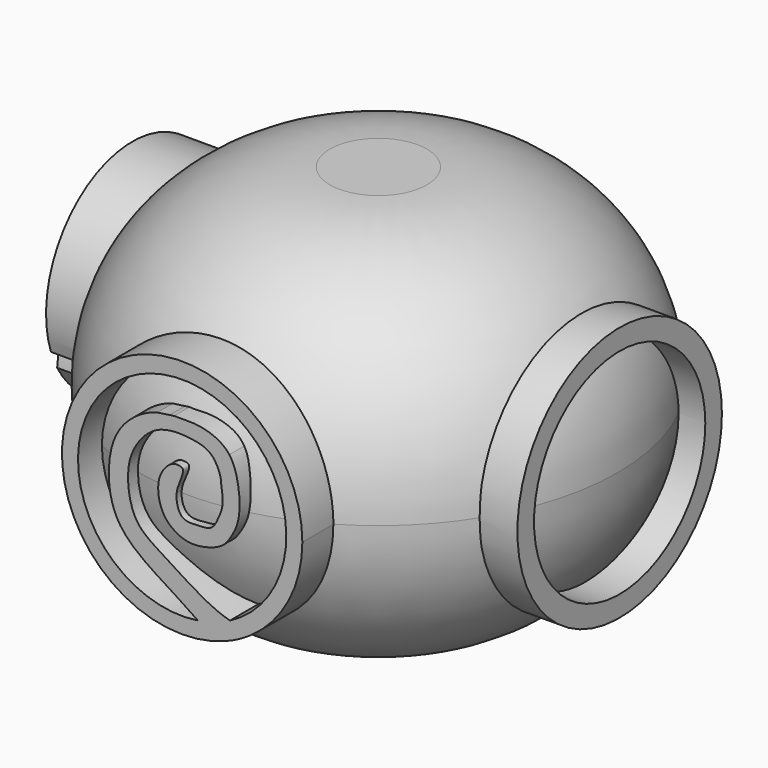
from build123d import *

# Parameters (mm, degrees)
F0_R      = 15.9252372122
F1_DEPTH  = 25.4
F2_R      = 12.69999
F5_DEPTH  = 4.826
F7_R      = 8.4966249318
F7_R_2    = 7.1160692684
F8_DEPTH  = 2.54
F11_DEPTH = 4.572


# Not quite as in the source:
# - a fillet or chamfer is up to 0.001 mm smaller than in the source, because OpenCascade refuses the exact size


with BuildPart() as f1:
    # F0 (on Top) → F1 (new body)
    with BuildSketch(Plane.XY):
        with Locations((-45.4665385187, 19.9958086014)):
            Circle(F0_R)
    extrude(amount=F1_DEPTH)

    # F2 (radius 12.7 in the source; OpenCascade refuses exactly that, so slightly less here)
    f2_edges = [f1.edges().sort_by_distance(p)[0] for p in [
        (-61.391776, 19.995809, 25.4),
        (-61.391776, 19.995809, 0),
    ]]
    fillet(f2_edges, radius=F2_R)

    # F4 (on offset) → F5 (join)
    with BuildSketch(Plane.XZ.offset(-8.4836)):
        with BuildLine():
            ThreePointArc((-40.8649766682, 6.1421600193), (-38.3567847687, 8.9987080945), (-37.4524912969, 12.6910172403))
            ThreePointArc((-37.4524912969, 12.6910172403), (-52.0299562046, 17.213182819), (-42.5712847542, 5.2346186709))
            add(Edge.make_bspline(
                [(-42.5712847542, 5.2346186709), (-43.2562301292, 5.1632855255), (-43.8271341007, 5.4728098032), (-44.3901814448, 5.8483672931)],
                knots=[0, 0, 0, 0, 0.0289246734, 0.0289246734, 0.0289246734, 0.0289246734], degree=3))
            ThreePointArc((-44.3901814448, 5.8483672931), (-47.5864163007, 19.273858808), (-42.2638656899, 6.5408232443))
            add(Edge.make_bspline(
                [(-42.2638656899, 6.5408232443), (-42.1252968592, 6.5032427239), (-41.4907211644, 6.3556006381), (-40.8609594383, 6.3320739122), (-40.8649397067, 6.1432060372), (-40.8649766682, 6.1421600193)],
                knots=[0.9364529104, 0.9364529104, 0.9364529104, 0.9364529104, 0.9431396587, 0.9671182162, 0.9672510998, 0.9672510998, 0.9672510998, 0.9672510998], degree=3))
        make_face()
        with BuildLine():
            add(Edge.make_bspline(
                [(-42.5712847542, 5.2346186709), (-43.2562301292, 5.1632855255), (-43.8271341007, 5.4728098032), (-44.3901814448, 5.8483672931)],
                knots=[0, 0, 0, 0, 0.0289246734, 0.0289246734, 0.0289246734, 0.0289246734], degree=3))
            ThreePointArc((-42.5712847542, 5.2346186709), (-41.6905903183, 5.6366094508), (-40.8649766682, 6.1421600193))
            add(Edge.make_bspline(
                [(-42.2638656899, 6.5408232443), (-42.1252968592, 6.5032427239), (-41.4907211644, 6.3556006381), (-40.8609594383, 6.3320739122), (-40.8649397067, 6.1432060372), (-40.8649766682, 6.1421600193)],
                knots=[0.9364529104, 0.9364529104, 0.9364529104, 0.9364529104, 0.9431396587, 0.9671182162, 0.9672510998, 0.9672510998, 0.9672510998, 0.9672510998], degree=3))
            add(Edge.make_bspline(
                [(-47.1967309713, 16.0708408803), (-47.833945179, 15.737785942), (-48.8182525875, 14.5189291184), (-49.1646515007, 12.723232856), (-48.7231346048, 10.0766539461), (-46.5014757479, 8.8666870456), (-44.362479312, 7.3659636528), (-42.8966973227, 6.7124501675), (-42.2638656899, 6.5408232443)],
                knots=[0.7259465401, 0.7259465401, 0.7259465401, 0.7259465401, 0.7606127871, 0.7926637022, 0.8295053434, 0.8661742116, 0.9059151204, 0.9364529104, 0.9364529104, 0.9364529104, 0.9364529104], degree=3))
            add(Edge.make_bspline(
                [(-47.1967309713, 16.0708408803), (-47.4068727664, 16.2299815358), (-47.3488955818, 16.8661833328), (-47.1007065866, 17.1431289381)],
                knots=[0.9666956427, 0.9666956427, 0.9666956427, 0.9666956427, 1, 1, 1, 1], degree=3))
            add(Edge.make_bspline(
                [(-44.3901814448, 5.8483672931), (-44.5553943922, 5.9585657701), (-45.5141446891, 6.6338183652), (-47.4284466831, 7.7490622806), (-50.1711333543, 9.8201576197), (-50.4844700957, 13.3229523668), (-49.6299716997, 15.7814837225), (-47.9901021889, 16.9115881053), (-47.1041946459, 17.1422263977), (-47.1007065866, 17.1431289381)],
                knots=[0.0289246734, 0.0289246734, 0.0289246734, 0.0289246734, 0.0374119358, 0.078379751, 0.1211195995, 0.1637398963, 0.201262983, 0.2402370067, 0.2403910313, 0.2403910313, 0.2403910313, 0.2403910313], degree=3))
        make_face()
        with BuildLine():
            Line((-46.2708222028, 17.2642140105), (-47.1007065866, 17.1431289381))
            add(Edge.make_bspline(
                [(-47.1967309713, 16.0708408803), (-47.4068727664, 16.2299815358), (-47.3488955818, 16.8661833328), (-47.1007065866, 17.1431289381)],
                knots=[0.9666956427, 0.9666956427, 0.9666956427, 0.9666956427, 1, 1, 1, 1], degree=3))
            add(Edge.make_bspline(
                [(-46.0861563159, 16.378780795), (-46.4744287147, 16.3423611219), (-46.8537935671, 16.2500851511), (-47.1967309713, 16.0708408803)],
                knots=[0.7072897797, 0.7072897797, 0.7072897797, 0.7072897797, 0.7259465401, 0.7259465401, 0.7259465401, 0.7259465401], degree=3))
            add(Edge.make_bspline(
                [(-45.0948283597, 16.3697992816), (-45.464682372, 16.4247345555), (-45.7256405416, 16.4961580256), (-46.0861563159, 16.378780795)],
                knots=[0.9002781283, 0.9002781283, 0.9002781283, 0.9002781283, 0.932237313, 0.932237313, 0.932237313, 0.932237313], degree=3))
            add(Edge.make_bspline(
                [(-44.3957208039, 16.2601374481), (-44.6158702618, 16.3124408527), (-44.8524488766, 16.3470509253), (-45.0948283597, 16.3697992816)],
                knots=[0.6796610012, 0.6796610012, 0.6796610012, 0.6796610012, 0.6914505544, 0.6914505544, 0.6914505544, 0.6914505544], degree=3))
            add(Edge.make_bspline(
                [(-43.5130821571, 15.8531471324), (-43.7611771188, 16.0794813325), (-44.0794329167, 16.1921687919), (-44.3957208039, 16.2601374481)],
                knots=[0.8588731101, 0.8588731101, 0.8588731101, 0.8588731101, 0.8821859457, 0.8821859457, 0.8821859457, 0.8821859457], degree=3))
            add(Edge.make_bspline(
                [(-43.2303411821, 15.5099774654), (-43.308568412, 15.6387488972), (-43.4002485883, 15.7545281531), (-43.5130821571, 15.8531471324)],
                knots=[0.6514894032, 0.6514894032, 0.6514894032, 0.6514894032, 0.6609197445, 0.6609197445, 0.6609197445, 0.6609197445], degree=3))
            add(Edge.make_bspline(
                [(-42.8716817835, 14.6470983211), (-42.889670745, 14.7810681302), (-43.0106875836, 15.1687829835), (-43.2303411821, 15.5099774654)],
                knots=[0.8213582789, 0.8213582789, 0.8213582789, 0.8213582789, 0.8487724957, 0.8487724957, 0.8487724957, 0.8487724957], degree=3))
            add(Edge.make_bspline(
                [(-42.7473448217, 13.3327562362), (-42.5489360646, 13.6694304686), (-42.7139026561, 14.1780855809), (-42.8716817835, 14.6470983211)],
                knots=[0.6061864187, 0.6061864187, 0.6061864187, 0.6061864187, 0.633248956, 0.633248956, 0.633248956, 0.633248956], degree=3))
            add(Edge.make_bspline(
                [(-45.8053322551, 12.8501367365), (-45.8093263418, 12.8122668097), (-45.8413164894, 12.3818324616), (-45.6203435887, 11.3296711054), (-44.4116511567, 11.4223345987), (-43.4304605186, 11.4348524949), (-43.0168487392, 12.3019583085), (-42.7579044115, 12.8988792839), (-42.7473448217, 13.3327562362)],
                knots=[0.6095974703, 0.6095974703, 0.6095974703, 0.6095974703, 0.6131012679, 0.6484424203, 0.6812370159, 0.7120003196, 0.7412503817, 0.7750597441, 0.7750597441, 0.7750597441, 0.7750597441], degree=3))
            add(Edge.make_bspline(
                [(-46.9431591796, 13.3920403221), (-46.6170833207, 13.2896622962), (-46.1951615295, 13.0406467356), (-45.8053322533, 12.8501367368)],
                knots=[0.525020717, 0.525020717, 0.525020717, 0.525020717, 0.5437775346, 0.5437775346, 0.5437775346, 0.5437775346], degree=3))
            add(Edge.make_bspline(
                [(-46.6405600309, 11.2791918218), (-46.8188770014, 11.5589204984), (-47.0514918647, 12.2118560679), (-47.0574274651, 13.0208637155), (-46.9431591668, 13.3920403182)],
                knots=[0.4105162826, 0.4105162826, 0.4105162826, 0.4105162826, 0.443347012, 0.4751192472, 0.4751192472, 0.4751192472, 0.4751192472], degree=3))
            add(Edge.make_bspline(
                [(-42.3247402359, 11.2555950961), (-42.8781920964, 10.9758512708), (-44.4977595803, 10.7330555799), (-46.0535324043, 10.9504098268), (-46.6405600309, 11.2791918218)],
                knots=[0.3989417799, 0.3989417799, 0.3989417799, 0.3989417799, 0.4275411211, 0.4641051357, 0.4641051357, 0.4641051357, 0.4641051357], degree=3))
            add(Edge.make_bspline(
                [(-42.3058085475, 16.2334536485), (-42.1569506996, 16.0353754741), (-41.7333334223, 15.2253788281), (-41.4388592615, 12.7640497149), (-42.0522446801, 11.6751077875), (-42.2999784205, 11.2925363615), (-42.3247402359, 11.2555950961)],
                knots=[0.1522198962, 0.1522198962, 0.1522198962, 0.1522198962, 0.1747765971, 0.2274955076, 0.2672672634, 0.2716522518, 0.2716522518, 0.2716522518, 0.2716522518], degree=3))
            add(Edge.make_bspline(
                [(-46.2708222028, 17.2642140105), (-45.6445014658, 17.2925560348), (-44.2389552439, 17.077746614), (-42.872279274, 16.6593578413), (-42.3058085475, 16.2334536485)],
                knots=[0.2524315128, 0.2524315128, 0.2524315128, 0.2524315128, 0.2793694764, 0.311616256, 0.311616256, 0.311616256, 0.311616256], degree=3))
        make_face()
        with BuildLine():
            Line((-45.9774620831, 17.3070169985), (-46.2708222028, 17.2642140105))
            add(Edge.make_bspline(
                [(-46.2708222028, 17.2642140105), (-45.6445014658, 17.2925560348), (-44.2389552439, 17.077746614), (-42.872279274, 16.6593578413), (-42.3058085475, 16.2334536485)],
                knots=[0.2524315128, 0.2524315128, 0.2524315128, 0.2524315128, 0.2793694764, 0.311616256, 0.311616256, 0.311616256, 0.311616256], degree=3))
            add(Edge.make_bspline(
                [(-45.9774620831, 17.3070169985), (-45.5494373055, 17.2799973839), (-44.7758297546, 17.3738463633), (-43.49110531, 17.1184031548), (-42.7278625526, 16.7041163227), (-42.3951108877, 16.3522840949), (-42.3058085475, 16.2334536485)],
                knots=[0.0341981308, 0.0341981308, 0.0341981308, 0.0341981308, 0.069641458, 0.1058900262, 0.1386877499, 0.1522198962, 0.1522198962, 0.1522198962, 0.1522198962], degree=3))
        make_face()
        with BuildLine():
            add(Edge.make_bspline(
                [(-45.0948283597, 16.3697992816), (-45.464682372, 16.4247345555), (-45.7256405416, 16.4961580256), (-46.0861563159, 16.378780795)],
                knots=[0.9002781283, 0.9002781283, 0.9002781283, 0.9002781283, 0.932237313, 0.932237313, 0.932237313, 0.932237313], degree=3))
            add(Edge.make_bspline(
                [(-45.0948283597, 16.3697992816), (-45.0966809644, 16.3699731565), (-45.4223765571, 16.4004136903), (-45.7583959897, 16.409524479), (-46.0861563159, 16.378780795)],
                knots=[0.6914505544, 0.6914505544, 0.6914505544, 0.6914505544, 0.6915406668, 0.7072897797, 0.7072897797, 0.7072897797, 0.7072897797], degree=3))
        make_face()
        with BuildLine():
            add(Edge.make_bspline(
                [(-42.3247402359, 11.2555950961), (-42.4776427693, 11.027485285), (-42.894888659, 10.5340277588), (-44.7556014252, 10.0274615865), (-45.9839159094, 10.5372886721), (-46.4706109355, 11.0125899643), (-46.6405600309, 11.2791918218)],
                knots=[0.2716522518, 0.2716522518, 0.2716522518, 0.2716522518, 0.2987292579, 0.3426957054, 0.3792261998, 0.4105162826, 0.4105162826, 0.4105162826, 0.4105162826], degree=3))
            add(Edge.make_bspline(
                [(-42.3247402359, 11.2555950961), (-42.8781920964, 10.9758512708), (-44.4977595803, 10.7330555799), (-46.0535324043, 10.9504098268), (-46.6405600309, 11.2791918218)],
                knots=[0.3989417799, 0.3989417799, 0.3989417799, 0.3989417799, 0.4275411211, 0.4641051357, 0.4641051357, 0.4641051357, 0.4641051357], degree=3))
        make_face()
        with BuildLine():
            add(Edge.make_bspline(
                [(-46.9431591668, 13.3920403182), (-46.9256835853, 13.4488060798), (-46.7624729448, 13.902042998), (-46.2074002547, 14.5211631721), (-45.7135851079, 14.5313217994), (-45.2677448497, 14.4421108974), (-45.5683048416, 13.6337326515), (-45.773191525, 13.1548790117), (-45.8053322551, 12.8501367365)],
                knots=[0.4751192472, 0.4751192472, 0.4751192472, 0.4751192472, 0.4799783226, 0.5143472841, 0.5362166132, 0.5540123445, 0.5814021355, 0.6095974703, 0.6095974703, 0.6095974703, 0.6095974703], degree=3))
            add(Edge.make_bspline(
                [(-46.9431591796, 13.3920403221), (-46.6170833207, 13.2896622962), (-46.1951615295, 13.0406467356), (-45.8053322533, 12.8501367368)],
                knots=[0.525020717, 0.525020717, 0.525020717, 0.525020717, 0.5437775346, 0.5437775346, 0.5437775346, 0.5437775346], degree=3))
        make_face()
        with BuildLine():
            add(Edge.make_bspline(
                [(-42.7473448217, 13.3327562362), (-42.5489360646, 13.6694304686), (-42.7139026561, 14.1780855809), (-42.8716817835, 14.6470983211)],
                knots=[0.6061864187, 0.6061864187, 0.6061864187, 0.6061864187, 0.633248956, 0.633248956, 0.633248956, 0.633248956], degree=3))
            add(Edge.make_bspline(
                [(-42.7473448217, 13.3327562362), (-42.7363601295, 13.784099978), (-42.9046292502, 14.540415439), (-42.8643796294, 14.5927167385), (-42.8716817835, 14.6470983211)],
                knots=[0.7750597441, 0.7750597441, 0.7750597441, 0.7750597441, 0.8102301858, 0.8213582789, 0.8213582789, 0.8213582789, 0.8213582789], degree=3))
        make_face()
    extrude(amount=F5_DEPTH)

    # F7 (on offset) → F8 (join)
    with BuildSketch(Plane.YZ.offset(-32.004)):
        with Locations((20.0373027474, 12.7005567774)):
            Circle(F7_R)
        with Locations((20.0373027474, 12.7005567774)):
            Circle(F7_R_2, mode=Mode.SUBTRACT)
    extrude(amount=F8_DEPTH)

    # F10 (on offset) → F11 (join)
    with BuildSketch(Plane.YZ.offset(-57.404)):
        with BuildLine():
            Line((22.2562696946, 3.7466434737), (22.2562696946, 7.3859567543))
            ThreePointArc((22.2562696946, 7.3859567543), (24.6805592334, 8.657320203), (26.4527660186, 10.7436633907))
            ThreePointArc((26.4527660186, 10.7436633907), (20.1951600611, 16.6159122004), (13.9375541036, 10.7436633907))
            ThreePointArc((13.9375541036, 10.7436633907), (15.718768807, 8.6501246298), (18.1561484933, 7.3793726368))
            Line((18.1561484933, 7.3793726368), (18.1561484933, 3.7466434737))
            Line((18.1561484933, 3.7466434737), (22.2562696946, 3.7466434737))
        make_face()
        with BuildLine():
            ThreePointArc((13.4226921152, 11.8802418148), (20.1951600611, 17.2898147506), (26.9676280071, 11.8802418148))
            ThreePointArc((26.9676280071, 11.8802418148), (20.1951600611, 21.4426958862), (13.4226921152, 11.8802418148))
        make_face()
    extrude(amount=-F11_DEPTH)


solid = f1.part
